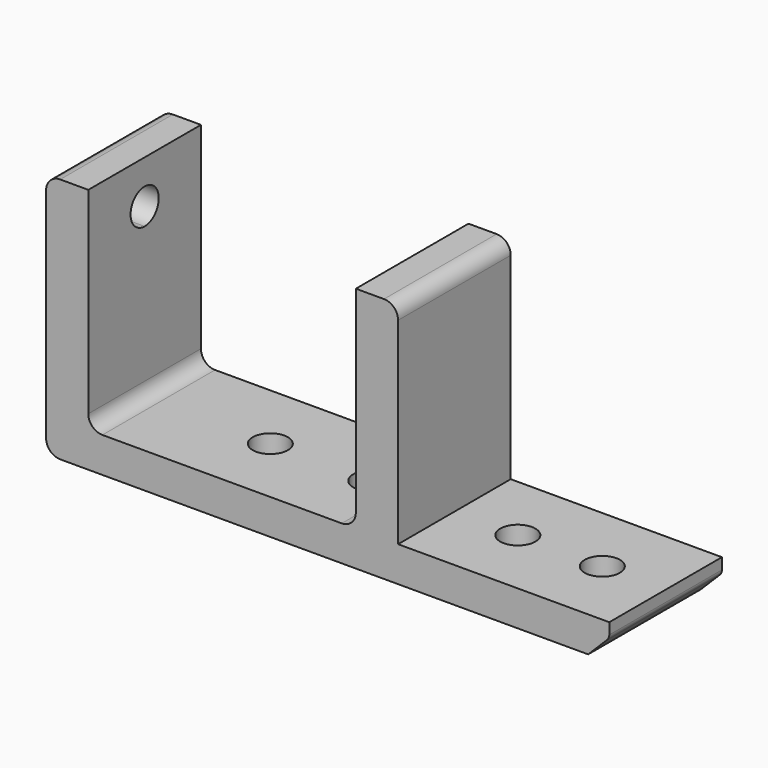
from build123d import *

# Parameters (mm, degrees)
F1_DEPTH = 35
F0_W     = 6
F0_H     = 20
F0_R     = 2.5
F0_W_2   = 30
F2_DEPTH = 5
F3_R     = 2
F4_SIZE  = 3
F5_R     = 1
F6_SIZE  = 2
F7_R     = 2
F9_DEPTH = 12.5


# Not quite as in the source:
# - a fillet or chamfer that OpenCascade refuses, or shapes differently, is made with other operations: its cross-section is extruded or revolved along the edge and cut away or added
# - a feature names something its author has since deleted; it is built from what else it names


with BuildPart() as f1:
    # F0 (on Top) → F1 (new body)
    with BuildSketch(Plane.XY):
        Polygon((-89.3438757165, 20.7090974661), (-89.3438757165, 30.7090974661), (-95.3438757165, 30.7090974661), (-95.3438757165, 10.7090974661), (-89.3438757165, 10.7090974661), align=None)
    extrude(amount=F1_DEPTH)



with BuildPart() as f1b:
    # F0 (on Top) → F1, piece 2 (new body)
    with BuildSketch(Plane.XY):
        with Locations((-48.3438757165, 20.7090974661)):
            Rectangle(F0_W, F0_H)
    extrude(amount=F1_DEPTH)


with BuildPart() as f1_1:
    add(f1.part)

    add(f1b.part)  # F2 merges F1b
    # F0 (on Top) → F2 (join)
    with BuildSketch(Plane.XY):
        Polygon((-51.3438757165, 30.7090974661), (-89.3438757165, 30.7090974661), (-89.3438757165, 20.7090974661), (-89.3438757165, 10.7090974661), (-51.3438757165, 10.7090974661), align=None)
        with Locations((-71.4934170246, 20.7090974661)):
            Circle(F0_R, mode=Mode.SUBTRACT)
        with Locations((-57.2206377983, 20.7090974661)):
            Circle(F0_R, mode=Mode.SUBTRACT)
        with Locations((-30.3438757165, 20.7090974661)):
            Rectangle(F0_W_2, F0_H)
        with Locations((-36.3354164958, 20.7090974661)):
            Circle(F0_R, mode=Mode.SUBTRACT)
        with Locations((-24.3354164958, 20.7090974661)):
            Circle(F0_R, mode=Mode.SUBTRACT)
    extrude(amount=F2_DEPTH)

    # F3
    f3_edges = [f1_1.edges().sort_by_distance(p)[0] for p in [
        (-89.343876, 20.709097, 5),
        (-51.343876, 20.709097, 5),
        (-45.343876, 20.709097, 35),
    ]]
    fillet(f3_edges, radius=F3_R)

    # F4
    f4_edges = [f1_1.edges().sort_by_distance(p)[0] for p in [
        (-15.343876, 20.709097, 0),
    ]]
    chamfer(f4_edges, length=F4_SIZE)

    # F5
    f5_edges = [f1_1.edges().sort_by_distance(p)[0] for p in [
        (-15.343876, 20.709097, 3),
    ]]
    fillet(f5_edges, radius=F5_R)

    # F6
    f6_edges = [f1_1.edges().sort_by_distance(p)[0] for p in [
        (-59.720638, 20.709097, 0),
        (-38.835416, 20.709097, 0),
        (-26.835416, 20.709097, 0),
        (-73.993417, 20.709097, 0),
    ]]
    chamfer(f6_edges, length=F6_SIZE)

    # F7
    f7_edges = [f1_1.edges().sort_by_distance(p)[0] for p in [
        (-95.343876, 20.709097, 35),
        (-95.343876, 20.709097, 0),
    ]]
    fillet(f7_edges, radius=F7_R)

    # F8 (on face) → F9 (cut, symmetric)
    with BuildSketch(Plane(origin=(-95.3438757165, 0, 0), x_dir=(0, -1, 0), z_dir=(-1, 0, 0))):
        with BuildLine():
            ThreePointArc((-18.2090974661, 28.8686309451), (-18.9413305132, 30.636397898), (-20.7090974661, 31.3686309451))
            Line((-20.7090974661, 31.3686309451), (-20.7090974661, 26.3686309451))
            ThreePointArc((-20.7090974661, 26.3686309451), (-18.9413305132, 27.1008639921), (-18.2090974661, 28.8686309451))
        make_face()
        with BuildLine():
            Line((-20.7090974661, 26.3686309451), (-20.7090974661, 31.3686309451))
            ThreePointArc((-20.7090974661, 31.3686309451), (-23.2090974661, 28.8686309451), (-20.7090974661, 26.3686309451))
        make_face()
    extrude(amount=F9_DEPTH, both=True, mode=Mode.SUBTRACT)

    # F10: chamfer of 2 on 1 edges, made by hand

    # F10_s1 → F10_t2 (revolve, cut)
    with BuildSketch(Plane.XY.offset(28.8686309451)):
        Polygon((-95.3438757165, 16.2090974661), (-93.3438757165, 18.2090974661), (-95.3438757165, 18.2090974661), align=None)
    revolve(axis=Axis((-95.3438757165, 20.7090974661, 28.8686309451), (-1, 0, 0)), mode=Mode.SUBTRACT)


solid = f1_1.part
